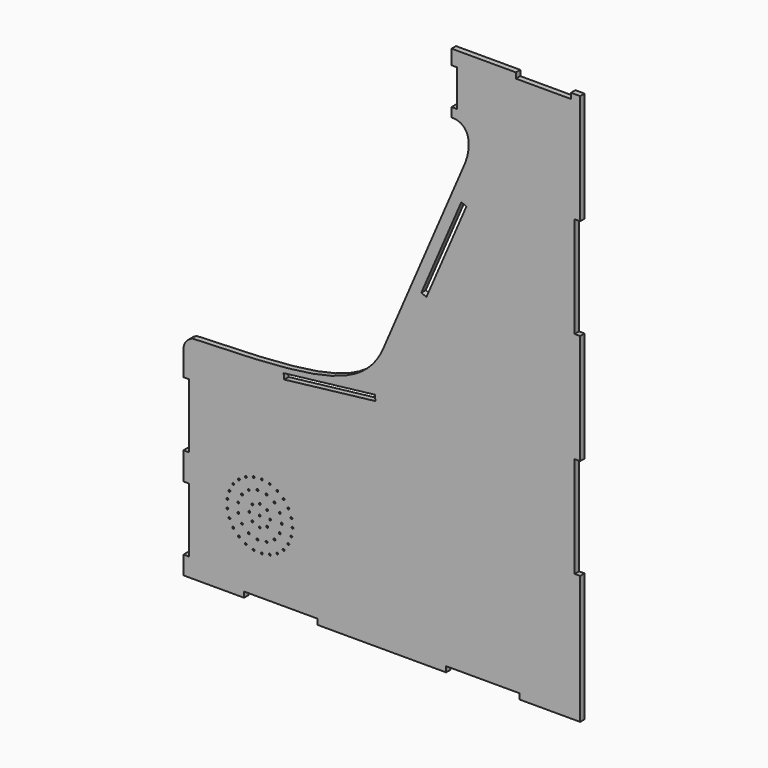
from build123d import *

# Parameters (mm, degrees)
F1_DEPTH = 3
F2_R     = 0.5
F3_DEPTH = 3


# Not quite as in the source:
# - a feature names something its author has since deleted; it is built from what else it names


with BuildPart() as f1:
    # F0 (on Front) → F1 (new body)
    with BuildSketch(Plane.XZ):
        with BuildLine():
            Line((0, 10), (0, 0))
            Line((0, 0), (33, 0))
            Line((33, 0), (33, 3))
            Line((33, 3), (73, 3))
            Line((73, 3), (73, 0))
            Line((73, 0), (143, 0))
            Line((143, 0), (143, 3))
            Line((143, 3), (183, 3))
            Line((183, 3), (183, 0))
            Line((183, 0), (216, 0))
            Line((216, 0), (216, 70))
            Line((216, 70), (213, 70))
            Line((213, 70), (213, 125))
            Line((213, 125), (216, 125))
            Line((216, 125), (216, 185))
            Line((216, 185), (213, 185))
            Line((213, 185), (213, 240))
            Line((213, 240), (216, 240))
            Line((216, 240), (216, 300))
            Line((216, 300), (211, 300))
            Line((211, 300), (211, 297))
            Line((211, 297), (181, 297))
            Line((181, 297), (181, 300))
            Line((181, 300), (176, 300))
            Line((176, 300), (174.706427271, 297))
            Line((174.706427271, 297), (161.7706999809, 267))
            Line((161.7706999809, 267), (152.9198643438, 246.4735105991))
            Line((152.9198643438, 246.4735105991), (108.8058184443, 144.1660525563))
            add(Edge.make_bspline(
                [(5.2380922861, 115.1536645525), (67.1986155562, 116.9837427001), (97.7651412543, 118.5609738259), (108.8058184443, 144.1660525563)],
                knots=[3.0455141627, 3.0455141627, 3.0455141627, 3.0455141627, 112.6470805172, 112.6470805172, 112.6470805172, 112.6470805172], degree=3))
            ThreePointArc((5.2380922861, 115.1536645525), (1.636924279, 112.8542013763), (0, 108.9075039192))
            Line((0, 108.9075039192), (0, 107.6488941908))
            Line((0, 107.6488941908), (0, 95))
            Line((0, 95), (3, 95))
            Line((3, 95), (3, 60))
            Line((3, 60), (0, 60))
            Line((0, 60), (0, 45))
            Line((0, 45), (3, 45))
            Line((3, 45), (3, 10))
            Line((3, 10), (0, 10))
        make_face()
        Polygon((54.8936169141, 111.7298124622), (54.5449186418, 114.7094784694), (104.2060187631, 120.5211163403), (104.5547170354, 117.541450333), align=None, mode=Mode.SUBTRACT)
        Polygon((129.52643753, 177.6246576271), (151.3037139596, 228.1296101695), (154.0585295529, 226.9417587279), (132.2812531233, 176.4368061855), align=None, mode=Mode.SUBTRACT)
        Polygon((146, 267), (161.7706999809, 267), (174.706427271, 297), (146, 297), (146, 292), (149, 292), (149, 272), (146, 272), align=None)
        Polygon((146, 297), (174.706427271, 297), (176, 300), (146, 300), align=None)
        with BuildLine():
            add(Edge.make_bspline(
                [(146, 267), (156.1105200986, 267), (157.3542433109, 256.7575376221), (152.9198643438, 246.4735105991)],
                knots=[0, 0, 0, 0, 21.6615163288, 21.6615163288, 21.6615163288, 21.6615163288], degree=3))
            Line((152.9198643438, 246.4735105991), (161.7706999809, 267))
            Line((161.7706999809, 267), (146, 267))
        make_face()
    extrude(amount=F1_DEPTH)

    # F2 (on face) → F3 (cut, through all)
    with BuildSketch(Plane.XZ.offset(3)):
        with Locations((41.5442730218, 42.1421974897)):
            Circle(F2_R)
        with Locations((47.2275130451, 42.1421974897)):
            Circle(F2_R)
        with Locations((53.483594209, 42.1421974897)):
            Circle(F2_R)
        with Locations((59.3261942267, 42.1421974897)):
            Circle(F2_R)
        with Locations((45.5629305814, 46.1608550493)):
            Circle(F2_R)
        with Locations((41.5442730218, 47.825437513)):
            Circle(F2_R)
        with Locations((37.5256154622, 46.1608550493)):
            Circle(F2_R)
        with Locations((35.8610329985, 42.1421974897)):
            Circle(F2_R)
        with Locations((37.5256154622, 38.1235399302)):
            Circle(F2_R)
        with Locations((41.5442730218, 36.4589574665)):
            Circle(F2_R)
        with Locations((45.5629305814, 38.1235399302)):
            Circle(F2_R)
        with Locations((52.4513856597, 46.99835691)):
            Circle(F2_R)
        with Locations((49.5332382473, 51.0148422497)):
            Circle(F2_R)
        with Locations((45.2337261699, 53.4971667049)):
            Circle(F2_R)
        with Locations((40.2962741256, 54.0161138262)):
            Circle(F2_R)
        with Locations((35.5746124282, 52.4819529418)):
            Circle(F2_R)
        with Locations((31.8851592801, 49.1599544059)):
            Circle(F2_R)
        with Locations((29.8658546482, 44.624521945)):
            Circle(F2_R)
        with Locations((29.8658546482, 39.6598730345)):
            Circle(F2_R)
        with Locations((31.8851592801, 35.1244405735)):
            Circle(F2_R)
        with Locations((35.5746124282, 31.8024420377)):
            Circle(F2_R)
        with Locations((40.2962741256, 30.2682811533)):
            Circle(F2_R)
        with Locations((45.2337261699, 30.7872282745)):
            Circle(F2_R)
        with Locations((49.5332382473, 33.2695527298)):
            Circle(F2_R)
        with Locations((52.4513856597, 37.2860380695)):
            Circle(F2_R)
        with Locations((58.7675424734, 46.5643814678)):
            Circle(F2_R)
        with Locations((57.1266893577, 50.7087033628)):
            Circle(F2_R)
        with Locations((54.5067357155, 54.3147601884)):
            Circle(F2_R)
        with Locations((51.0723028696, 57.1559701322)):
            Circle(F2_R)
        with Locations((47.0391888668, 59.053809524)):
            Circle(F2_R)
        with Locations((42.6608090925, 59.8890301351)):
            Circle(F2_R)
        with Locations((38.2122732505, 59.6091519828)):
            Circle(F2_R)
        with Locations((33.9730992085, 58.2317608408)):
            Circle(F2_R)
        with Locations((30.2096498619, 55.8434032602)):
            Circle(F2_R)
        with Locations((27.1583965743, 52.5941485314)):
            Circle(F2_R)
        with Locations((25.0110608115, 48.6881592792)):
            Circle(F2_R)
        with Locations((23.9025675767, 44.3708631733)):
            Circle(F2_R)
        with Locations((23.9025675767, 39.9135318061)):
            Circle(F2_R)
        with Locations((25.0110608115, 35.5962357003)):
            Circle(F2_R)
        with Locations((27.1583965743, 31.690246448)):
            Circle(F2_R)
        with Locations((30.2096498619, 28.4409917193)):
            Circle(F2_R)
        with Locations((33.9730992085, 26.0526341387)):
            Circle(F2_R)
        with Locations((38.2122732505, 24.6752429966)):
            Circle(F2_R)
        with Locations((42.6608090925, 24.3953648444)):
            Circle(F2_R)
        with Locations((47.0391888668, 25.2305854555)):
            Circle(F2_R)
        with Locations((51.0723028696, 27.1284248473)):
            Circle(F2_R)
        with Locations((54.5067357155, 29.969634791)):
            Circle(F2_R)
        with Locations((57.1266893577, 33.5756916167)):
            Circle(F2_R)
        with Locations((58.7675424734, 37.7200135117)):
            Circle(F2_R)
    extrude(amount=-F3_DEPTH, mode=Mode.SUBTRACT)


solid = f1.part
